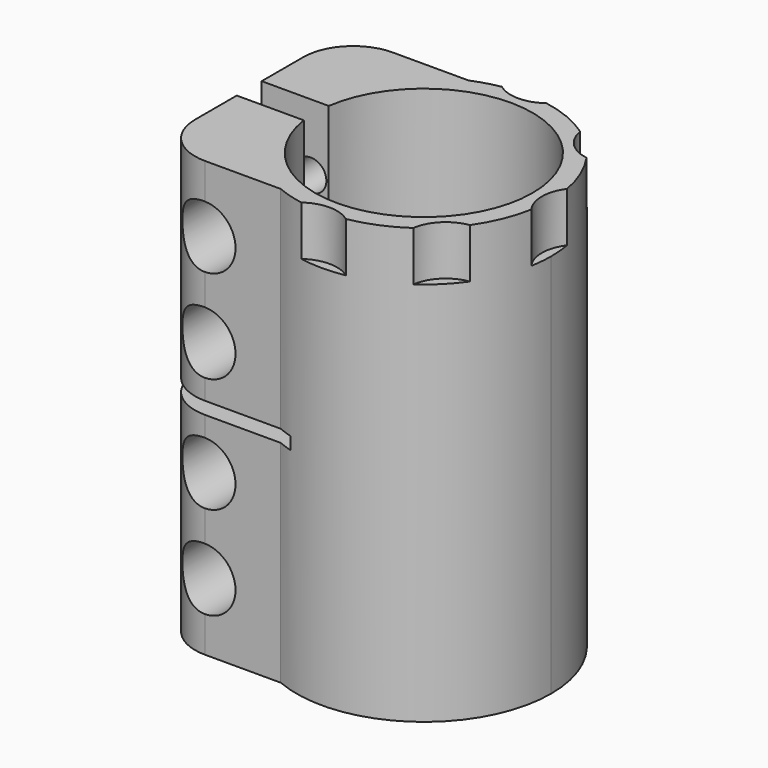
from build123d import *

# Parameters (mm, degrees)
F1_DEPTH       = 35
F3_D           = 5
F3_START       = 1.820508
F3_CBORE_D     = 10
F3_CBORE_DEPTH = 8
F4_W           = 22.4
F4_H           = 2
F5_DEPTH       = 25
F6_R           = 6
F7_DEPTH       = 8


with BuildPart() as f1:
    # F0 (on Top) → F1 (new body, symmetric)
    with BuildSketch(Plane.XY):
        with BuildLine():
            ThreePointArc((17.5, 0), (1.257552, -17.454758), (-17.319264, -2.508603))
            Line((-17.319264, -2.508603), (-28.119264, -2.508603))
            Line((-28.119264, -2.508603), (-28.119264, -10.908603))
            ThreePointArc((-28.119264, -10.908603), (-25.776118, -16.565457), (-20.119264, -18.908603))
            Line((-20.119264, -18.908603), (-7.919264, -18.908603))
            ThreePointArc((-7.919264, -18.908603), (11.355727, -17.067439), (20.5, 0))
            Line((20.5, 0), (17.5, 0))
        make_face()
        with BuildLine():
            ThreePointArc((-17.319264, 2.508603), (1.257552, 17.454758), (17.5, 0))
            Line((17.5, 0), (20.5, 0))
            ThreePointArc((20.5, 0), (11.355727, 17.067439), (-7.919264, 18.908603))
            Line((-7.919264, 18.908603), (-20.119264, 18.908603))
            ThreePointArc((-20.119264, 18.908603), (-25.776118, 16.565457), (-28.119264, 10.908603))
            Line((-28.119264, 10.908603), (-28.119264, 2.508603))
            Line((-28.119264, 2.508603), (-17.319264, 2.508603))
        make_face()
    extrude(amount=F1_DEPTH, both=True)

    # F3 (through all)
    # its depths count from where the whole tool has entered the part; down to there all is cleared
    with Locations(Plane.XZ.offset(18.908603).offset(-F3_START)):
        with Locations((-20.2, 24.25), (-20.2, 9.25), (-20.2, -9.25), (-20.2, -24.25)):
            CounterBoreHole(F3_D / 2, F3_CBORE_D / 2, F3_CBORE_DEPTH)

    # F4 (on Front) → F5 (cut, symmetric)
    with BuildSketch(Plane.XZ):
        with Locations((-16.919264, 0)):
            Rectangle(F4_W, F4_H)
    extrude(amount=F5_DEPTH, both=True, mode=Mode.SUBTRACT)

    # F6 (on face) → F7 (cut)
    with BuildSketch(Plane.XY.offset(35)):
        with Locations((0, -25)):
            Circle(F6_R)
        with Locations((17.67767, -17.67767)):
            Circle(F6_R)
        with Locations((25, 0)):
            Circle(F6_R)
        with Locations((17.67767, 17.67767)):
            Circle(F6_R)
        with Locations((0, 25)):
            Circle(F6_R)
    extrude(amount=-F7_DEPTH, mode=Mode.SUBTRACT)


solid = f1.part
